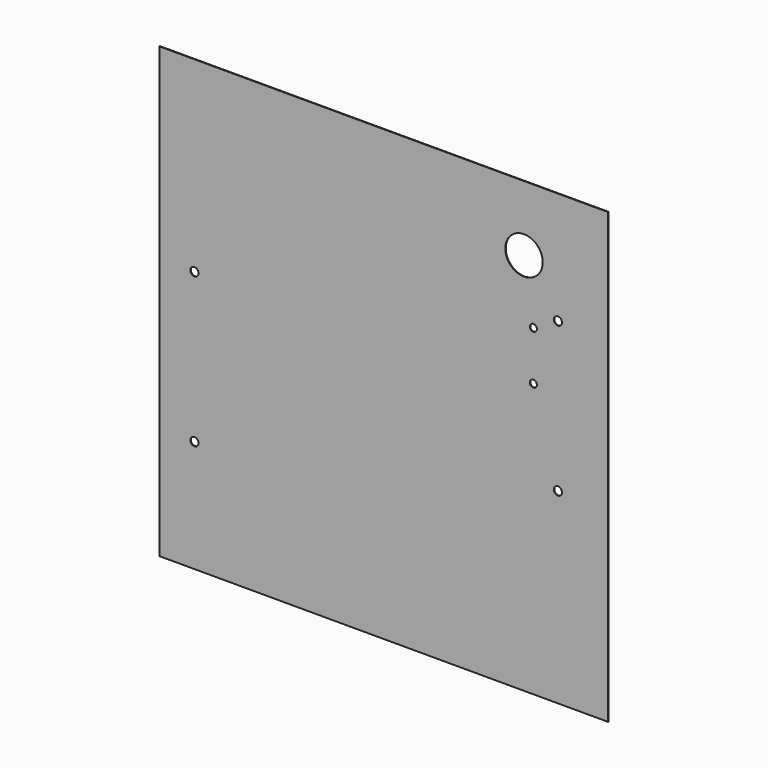
from build123d import *

# Parameters (mm, degrees)
F0_W     = 609.6
F0_H     = 609.6
F1_DEPTH = 0.79375
F2_R     = 5.55625
F3_DEPTH = 25.4
F4_R     = 25.4
F4_R_2   = 4.7625
F5_DEPTH = 25.4


# Not quite as in the source:
# - a feature names something its author has since deleted; it is built from what else it names


with BuildPart() as f1:
    # F0 (on Front) → F1 (new body)
    with BuildSketch(Plane.XZ):
        with Locations((304.8, 304.8)):
            Rectangle(F0_W, F0_H)
    extrude(amount=F1_DEPTH)

    # F2 (on face) → F3 (cut)
    with BuildSketch(Plane.XZ.offset(0.79375)):
        with Locations((47.625, 355.6)):
            Circle(F2_R)
        with Locations((47.625, 152.4)):
            Circle(F2_R)
        with Locations((541.3375, 254)):
            Circle(F2_R)
        with Locations((541.3375, 457.2)):
            Circle(F2_R)
    extrude(amount=-F3_DEPTH, mode=Mode.SUBTRACT)

    # F4 (on face) → F5 (cut)
    with BuildSketch(Plane.XZ.offset(0.79375)):
        with Locations((495.3, 520.7)):
            Circle(F4_R)
        with Locations((508, 438.15)):
            Circle(F4_R_2)
        with Locations((508, 371.475)):
            Circle(F4_R_2)
    extrude(amount=-F5_DEPTH, mode=Mode.SUBTRACT)


solid = f1.part
